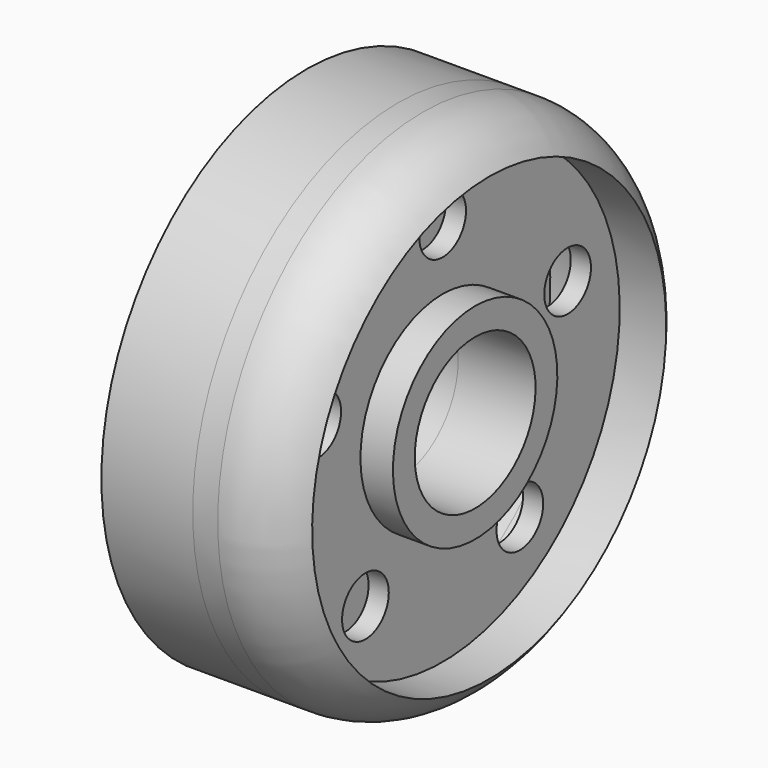
from build123d import *

# Parameters (mm, degrees)
F2_R     = 6.2476650757
F3_DEPTH = 25


# Not quite as in the source:
# - a fillet or chamfer that OpenCascade refuses, or shapes differently, is made with other operations: its cross-section is extruded or revolved along the edge and cut away or added


with BuildPart() as f1:
    # F0 (on Front) → F1 (revolve)
    with BuildSketch(Plane.XZ):
        Polygon((19.546540454, 54.8806712031), (0, 54.8806712031), (0, 47.3627708852), (5.2625308745, 47.3627708852), (5.2625308745, 21.989857778), (0, 21.989857778), (0, 16.1634851247), (16.5393799543, 16.1634851247), (16.5393799543, 21.989857778), (9.5853218809, 21.989857778), (9.5853218809, 47.3627708852), (19.546540454, 47.3627708852), align=None)
    revolve(axis=Axis((6.3902153634, 0, 0), (1, 0, 0)))

    # F2 (on face) → F3 (cut)
    with BuildSketch(Plane.YZ.offset(9.5853218809)):
        with Locations((0, 35.1461842656)):
            Circle(F2_R)
        with Locations((-33.4260075687, 10.8607682255)):
            Circle(F2_R)
        with Locations((33.4260075687, 10.8607682255)):
            Circle(F2_R)
        with Locations((20.6584087857, -28.4338603583)):
            Circle(F2_R)
        with Locations((-20.6584087857, -28.4338603583)):
            Circle(F2_R)
    extrude(amount=-F3_DEPTH, mode=Mode.SUBTRACT)


with BuildPart() as f4_1:
    # F4: instance of F1
    add(f1.part.mirror(Plane.YZ))


with BuildPart() as f1_1:
    add(f1.part)

    # F5: fillet of radius 17.1698868556 on 1 edges, made by hand

    # F5_s1 → F5_t2 (revolve, cut)
    with BuildSketch(Plane.XZ):
        with BuildLine():
            ThreePointArc((5.3463936058, 54.8806712031), (13.3801193246, 52.8852453168), (19.546540454, 47.3627708852))
            Line((19.546540454, 47.3627708852), (19.830543391, 47.555810616))
            ThreePointArc((19.830543391, 47.555810616), (19.8899381911, 51.1217210442), (19.8899381911, 54.8806712031))
            Line((19.8899381911, 54.8806712031), (19.546540454, 55.2240689402))
            Line((19.546540454, 55.2240689402), (5.3463936058, 55.2240689402))
            Line((5.3463936058, 55.2240689402), (5.3463936058, 54.8806712031))
        make_face()
    revolve(axis=Axis((19.546540454, 0, 0), (1, 0, 0)), mode=Mode.SUBTRACT)


solid = Compound([f4_1.part, f1_1.part])
